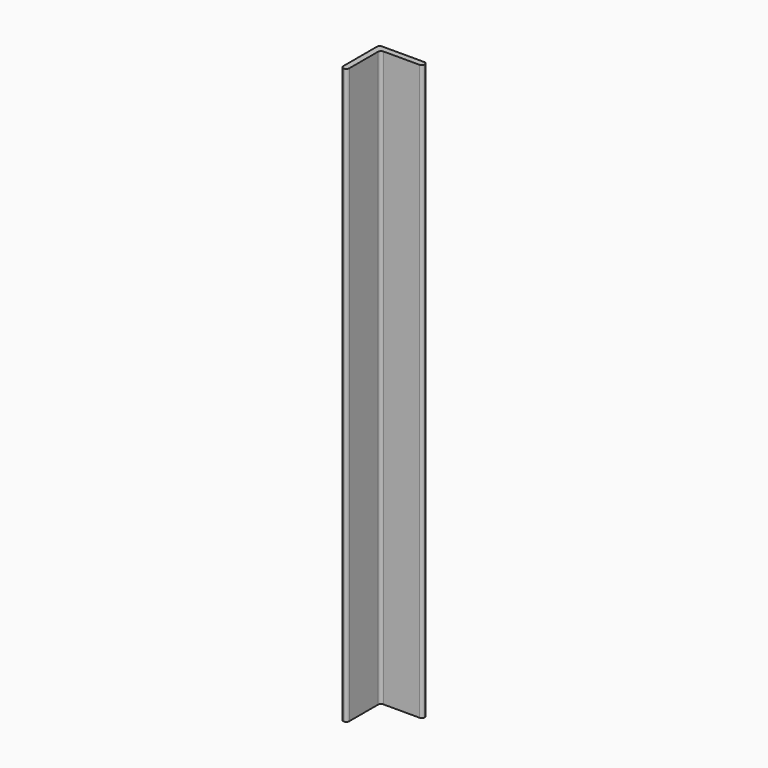
from build123d import *

# Parameters (mm, degrees)
F1_DEPTH = 609.6
F2_R     = 3.17499


# Not quite as in the source:
# - a fillet or chamfer is up to 0.001 mm smaller than in the source, because OpenCascade refuses the exact size


with BuildPart() as f1:
    # F0 (on Top) → F1 (new body)
    with BuildSketch(Plane.XY):
        Polygon((0, 22.2098889381), (0, -28.5901110619), (6.35, -28.5901110619), (6.35, 15.8598889381), (50.8, 15.8598889381), (50.8, 22.2098889381), align=None)
    extrude(amount=F1_DEPTH)

    # F2 (radius 3.175 in the source; OpenCascade refuses exactly that, so slightly less here)
    f2_edges = [f1.edges().sort_by_distance(p)[0] for p in [
        (0, -28.590111, 304.8),
        (6.35, -28.590111, 304.8),
        (6.35, 15.859889, 304.8),
        (50.8, 15.859889, 304.8),
        (50.8, 22.209889, 304.8),
        (0, 22.209889, 304.8),
    ]]
    fillet(f2_edges, radius=F2_R)


solid = f1.part
